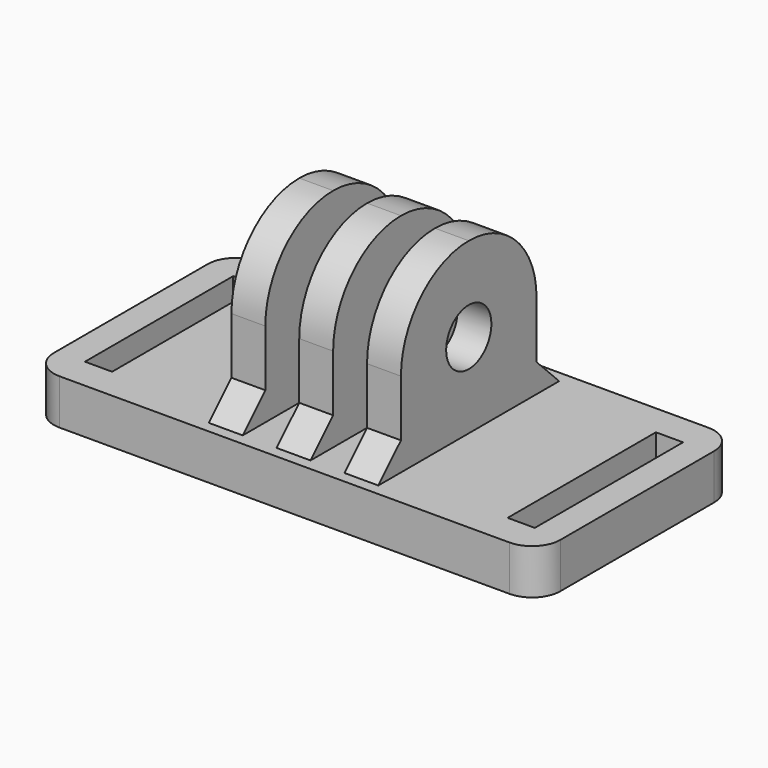
from build123d import *

# Parameters (mm, degrees)
F0_W     = 2.4047140032
F0_H     = 16.4
F0_W_2   = 3
F0_H_2   = 7.5
F0_W_3   = 1.5
F1_DEPTH = 4
F2_DEPTH = 19
F3_R     = 7.49999
F4_R     = 2.5
F5_DEPTH = 29.9057140032
F6_SIZE  = 2.5
F7_R     = 2.5


# Not quite as in the source:
# - a fillet or chamfer is up to 0.001 mm smaller than in the source, because OpenCascade refuses the exact size
# - a feature names something its author has since deleted; it is built from what else it names


with BuildPart() as f1:
    # F0 (on Top) → F1 (new body)
    with BuildSketch(Plane.XY):
        Polygon((-5.6430239742, 11), (-22.4047140032, 11), (-22.4047140032, -11), (22.4047140032, -11), (22.4047140032, 11), (5.6430239742, 11), (0, 11), align=None)
        with Locations((-18.7023570016, 0)):
            Rectangle(F0_W, F0_H, mode=Mode.SUBTRACT)
        Polygon((-1.5, 7.5), (0, 7.5), (1.5, 7.5), (4.5, 7.5), (7.5, 7.5), (7.5, -7.5), (4.5, -7.5), (4.5, 0), (1.5, 0), (1.5, -7.5), (-1.5, -7.5), (-1.5, 0), (-4.5, 0), (-4.5, -7.5), (-7.5, -7.5), (-7.5, 7.5), (-4.5, 7.5), align=None, mode=Mode.SUBTRACT)
        with Locations((18.7023570016, 0)):
            Rectangle(F0_W, F0_H, mode=Mode.SUBTRACT)
        Polygon((-4.5, 0), (-4.5, 7.5), (-7.5, 7.5), (-7.5, -7.5), (-4.5, -7.5), align=None)
        with Locations((-3, 3.75)):
            Rectangle(F0_W_2, F0_H_2)
        with Locations((-0.75, 3.75)):
            Rectangle(F0_W_3, F0_H_2)
        with Locations((0.75, 3.75)):
            Rectangle(F0_W_3, F0_H_2)
        Polygon((1.5, 0), (0, 0), (-1.5, 0), (-1.5, -7.5), (1.5, -7.5), align=None)
        with Locations((3, 3.75)):
            Rectangle(F0_W_2, F0_H_2)
        Polygon((7.5, 7.5), (4.5, 7.5), (4.5, 0), (4.5, -7.5), (7.5, -7.5), align=None)
    extrude(amount=F1_DEPTH)

    # F0 (on Top) → F2 (join)
    with BuildSketch(Plane.XY):
        Polygon((-4.5, 0), (-4.5, 7.5), (-7.5, 7.5), (-7.5, -7.5), (-4.5, -7.5), align=None)
        with Locations((-0.75, 3.75)):
            Rectangle(F0_W_3, F0_H_2)
        with Locations((0.75, 3.75)):
            Rectangle(F0_W_3, F0_H_2)
        Polygon((1.5, 0), (0, 0), (-1.5, 0), (-1.5, -7.5), (1.5, -7.5), align=None)
        Polygon((7.5, 7.5), (4.5, 7.5), (4.5, 0), (4.5, -7.5), (7.5, -7.5), align=None)
    extrude(amount=F2_DEPTH)

    # F3 (radius 7.5 in the source; OpenCascade refuses exactly that, so slightly less here)
    f3_edges = [f1.edges().sort_by_distance(p)[0] for p in [
        (-6, -7.5, 19),
        (0, -7.5, 19),
        (6, -7.5, 19),
        (6, 7.5, 19),
        (0, 7.5, 19),
        (-6, 7.5, 19),
    ]]
    fillet(f3_edges, radius=F3_R)

    # F4 (on face) → F5 (cut, through all)
    with BuildSketch(Plane(origin=(-7.5, 0, 0), x_dir=(0, -1, 0), z_dir=(-1, 0, 0))):
        with Locations((0, 11.5)):
            Circle(F4_R)
    extrude(amount=-F5_DEPTH, mode=Mode.SUBTRACT)

    # F6
    f6_edges = [f1.edges().sort_by_distance(p)[0] for p in [
        (-6, 7.5, 4),
        (0, 7.5, 4),
        (6, 7.5, 4),
        (-6, -7.5, 4),
        (0, -7.5, 4),
        (6, -7.5, 4),
    ]]
    chamfer(f6_edges, length=F6_SIZE)

    # F7
    f7_edges = [f1.edges().sort_by_distance(p)[0] for p in [
        (-22.404714, 11, 2),
        (-22.404714, -11, 2),
        (22.404714, -11, 2),
        (22.404714, 11, 2),
    ]]
    fillet(f7_edges, radius=F7_R)


solid = f1.part
